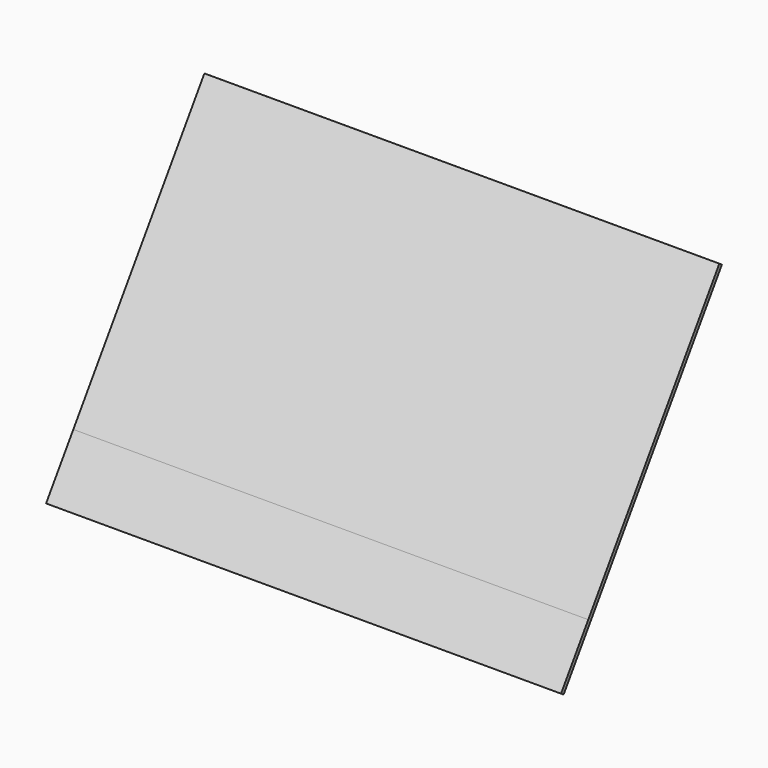
from build123d import *

# Parameters (mm, degrees)
F1_E1_W  = 1102.2678382234
F1_E1_H  = 9220.2
F1_E0_W  = 5304.66397145
F1_E0_H  = 9220.2
F2_DEPTH = 69.135625


with BuildPart() as f2:
    # F1_E1 (on explicit) + F1_E0 (on explicit) → F2 (new body)
    with BuildSketch(Plane(origin=(-4610.1, -2933.7, 6096), x_dir=(0, -0.5530416282, -0.8331536218), z_dir=(0, -0.8331536218, 0.5530416282))):
        with Locations((551.1339191117, 4610.1)):
            Rectangle(F1_E1_W, F1_E1_H)
    with BuildSketch(Plane(origin=(-4610.1, 0, 10515.6), x_dir=(0, -0.5530416282, -0.8331536218), z_dir=(0, -0.8331536218, 0.5530416282))):
        with Locations((2652.331985725, 4610.1)):
            Rectangle(F1_E0_W, F1_E0_H)
    extrude(amount=F2_DEPTH)


solid = f2.part
